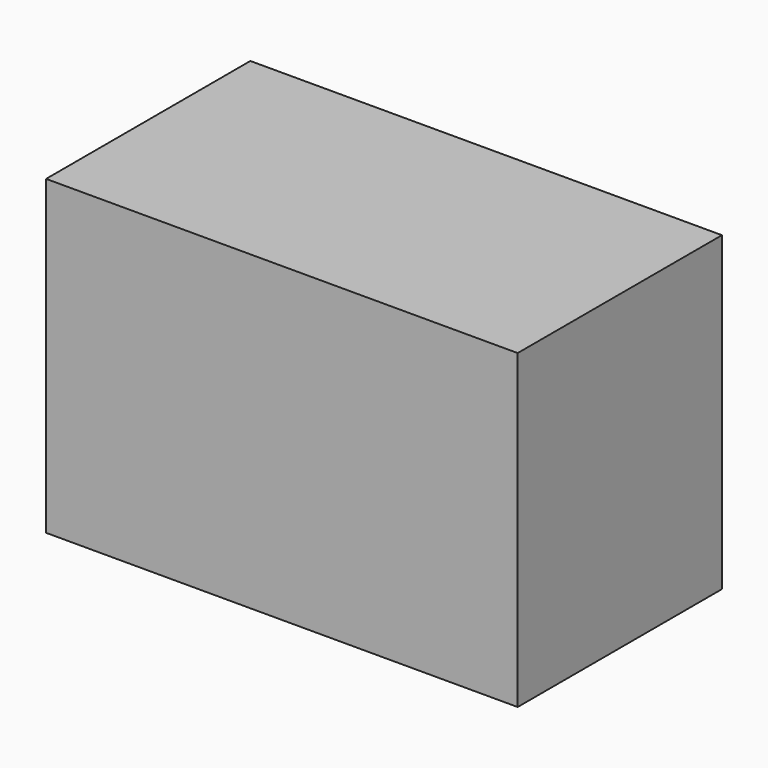
from build123d import *

# Parameters (mm, degrees)
F0_W     = 120.3951835632
F0_H     = 79.5549862087
F2_DEPTH = 65.1818728074


# Not quite as in the source:
# - the program builds the solid bodies; features that only make, move or delete a surface that nothing else refers to are left out


with BuildPart() as f2:
    # F0 (on Front) → F2 (new body)
    with BuildSketch(Plane.XZ):
        with Locations((0.388354063, -17.5738651305)):
            Rectangle(F0_W, F0_H)
    extrude(amount=-F2_DEPTH)


solid = f2.part
